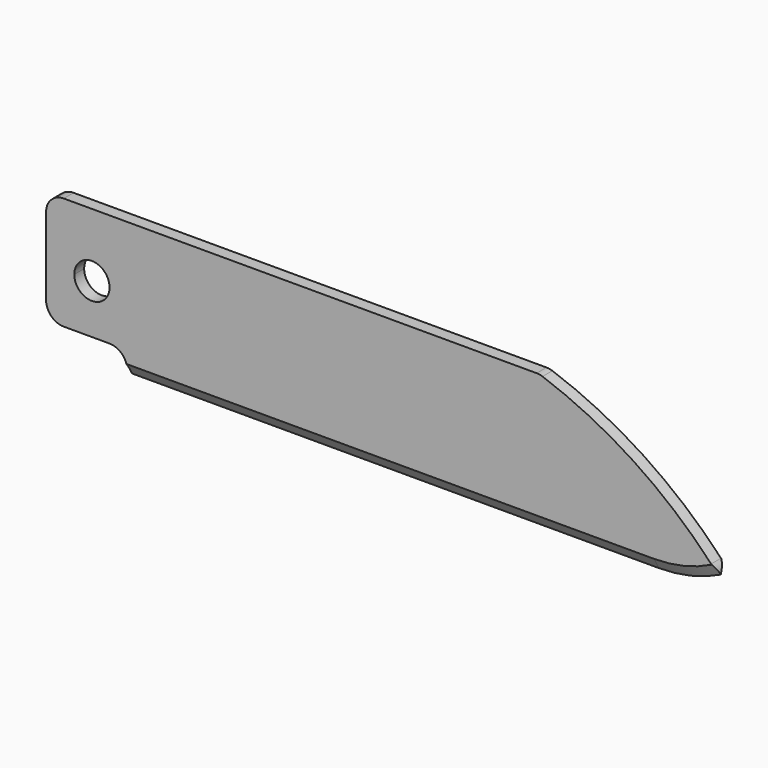
from build123d import *

# Parameters (mm, degrees)
F1_DEPTH    = 1.75
F2_F1_R     = 2.5
F2_F2_R     = 2.5
F3_T1_DEPTH = 45.6015639847
F4_T1_DEPTH = 79.2106511737
F4_T4_ANGLE = 38.8466581594
F4_T6_ANGLE = 38.8466581594


# Not quite as in the source:
# - a fillet or chamfer that OpenCascade refuses, or shapes differently, is made with other operations: its cross-section is extruded or revolved along the edge and cut away or added


with BuildPart() as f1:
    # F0 (on Front) → F1 (new body)
    with BuildSketch(Plane.XZ):
        with BuildLine():
            Line((-47.5, -6.25), (-36, -6.25))
            Line((-36, -6.25), (-36, 9.75))
            Line((-36, 9.75), (-41, 9.75))
            Line((-41, 9.75), (-41, 3.25))
            ThreePointArc((-41, 3.25), (-39.232233047, 2.517766953), (-38.5, 0.75))
            ThreePointArc((-38.5, 0.75), (-41, -1.75), (-43.5, 0.75))
            Line((-43.5, 0.75), (-47.5, 0.75))
            Line((-47.5, 0.75), (-47.5, -6.25))
        make_face()
        with BuildLine():
            Line((-36, -9.75), (47.5, -9.75))
            Line((47.5, -9.75), (47.5, -6.75))
            ThreePointArc((47.5, -6.75), (36.0462328118, 3.08520123), (22.5, 9.75))
            Line((22.5, 9.75), (-36, 9.75))
            Line((-36, 9.75), (-36, -6.25))
            Line((-36, -6.25), (-36, -9.75))
        make_face()
        with BuildLine():
            Line((-47.5, 9.75), (-47.5, 0.75))
            Line((-47.5, 0.75), (-43.5, 0.75))
            ThreePointArc((-43.5, 0.75), (-42.767766953, 2.517766953), (-41, 3.25))
            Line((-41, 3.25), (-41, 9.75))
            Line((-41, 9.75), (-47.5, 9.75))
        make_face()
    extrude(amount=F1_DEPTH)

    # F2: fillet of radius 2.5 on 5 edges, made by hand

    # F2_f1
    f2_f1_edges = [f1.edges().sort_by_distance(p)[0] for p in [
        (-36, -0.875, -6.25),
    ]]
    fillet(f2_f1_edges, radius=F2_F1_R)

    # F2_f2
    f2_f2_edges = [f1.edges().sort_by_distance(p)[0] for p in [
        (-47.5, -0.875, -6.25),
        (-47.5, -0.875, 9.75),
        (22.5, -0.875, 9.75),
        (47.5, -0.875, -6.75),
    ]]
    fillet(f2_f2_edges, radius=F2_F2_R)

    # F3: fillet of radius 20 on 1 edges, made by hand

    # F3_s2 → F3_t1 (cut)
    with BuildSketch(Plane.XZ.offset(-21.9257819924)):
        with BuildLine():
            ThreePointArc((38.7296872031, -9.75), (43.2302747659, -9.2370395799), (47.5, -7.7244711589))
            Line((47.5, -7.7244711589), (47.5, -9.75))
            Line((47.5, -9.75), (38.7296872031, -9.75))
        make_face()
    extrude(amount=F3_T1_DEPTH, mode=Mode.SUBTRACT)

    # F4: chamfer of 1 x 1.7320508076 on 4 edges, made by hand

    # F4_s2 → F4_t1 (cut)
    with BuildSketch(Plane.YZ.offset(-40.4809639706)):
        Polygon((-1.75, -8.0179491924), (-0.75, -9.75), (-1.75, -9.75), align=None)
        Polygon((0, -8.0179491924), (-1, -9.75), (0, -9.75), align=None)
    extrude(amount=F4_T1_DEPTH, mode=Mode.SUBTRACT)

    # F4_s3 → F4_t4 (revolve, cut)
    with BuildSketch(Plane(origin=(28.4995819615, 0, 22.9524885444), x_dir=(0, 1, 0), z_dir=(0.778827439, 0, 0.6272382484))):
        Polygon((0, -34.577709107), (-1, -36.3097599146), (0, -36.3097599146), align=None)
    revolve(axis=Axis((38.729687203, 0, 10.2499999998), (0, 1, 0)), revolution_arc=F4_T4_ANGLE, mode=Mode.SUBTRACT)

    # F4_s5 → F4_t6 (revolve, cut)
    with BuildSketch(Plane(origin=(28.4995819615, 0, 22.9524885444), x_dir=(0, 1, 0), z_dir=(0.778827439, 0, 0.6272382484))):
        Polygon((-1.75, -34.577709107), (-0.75, -36.3097599146), (-1.75, -36.3097599146), align=None)
    revolve(axis=Axis((38.729687203, -1.75, 10.2499999998), (0, 1, 0)), revolution_arc=F4_T6_ANGLE, mode=Mode.SUBTRACT)


solid = f1.part
